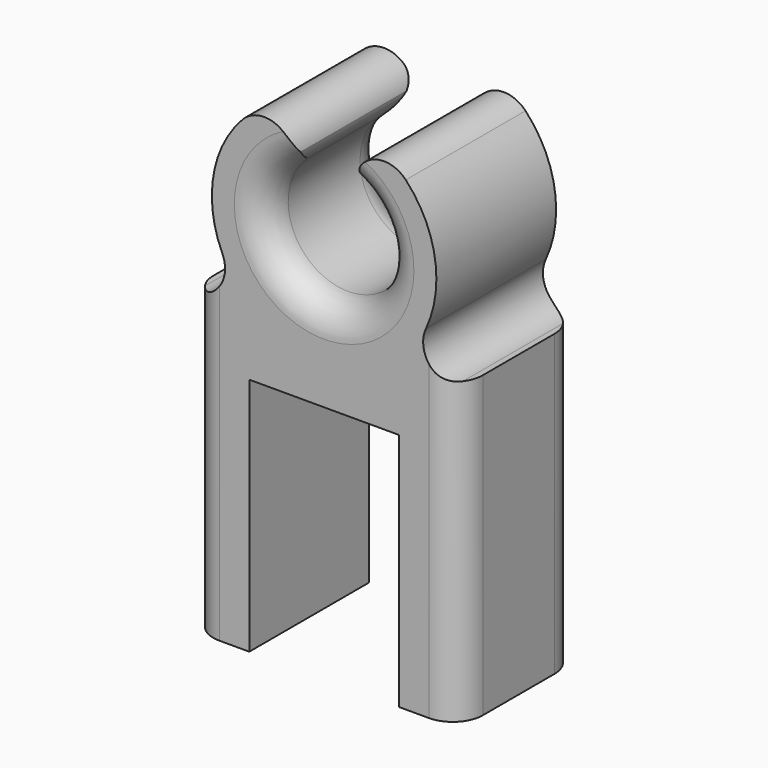
from build123d import *

# Parameters (mm, degrees)
F1_DEPTH    = 5
F2_R        = 7.5
F2_R_2      = 4
F3_DEPTH    = 5
F4_W        = 4
F4_H        = 10
F5_DEPTH    = 5.7
F6_T1_DEPTH = 10
F6_T3_DEPTH = 30.1640895286
F6_T5_DEPTH = 15.0401716993
F7_R        = 2
F8_T2_ANGLE = 359.64
F8_T4_ANGLE = 359.64


# Not quite as in the source:
# - a fillet or chamfer that OpenCascade refuses, or shapes differently, is made with other operations: its cross-section is extruded or revolved along the edge and cut away or added


with BuildPart() as f1:
    # F0 (on Front) → F1 (new body, symmetric)
    with BuildSketch(Plane.XZ):
        Polygon((-4, 0), (0, 0), (0, 16), (10, 16), (10, 0), (14, 0), (14, 20), (-4, 20), align=None)
    extrude(amount=F1_DEPTH, both=True)

    # F2 (on Front) → F3 (join, symmetric)
    with BuildSketch(Plane.XZ):
        with Locations((5, 26)):
            Circle(F2_R)
        with Locations((5, 26)):
            Circle(F2_R_2, mode=Mode.SUBTRACT)
    extrude(amount=F3_DEPTH, both=True)

    # F4 (on Front) → F5 (cut, symmetric)
    with BuildSketch(Plane.XZ):
        with Locations((5, 31.8401088891)):
            Rectangle(F4_W, F4_H)
    extrude(amount=F5_DEPTH, both=True, mode=Mode.SUBTRACT)

    # F6: fillet of radius 2 on 6 edges, made by hand

    # F6_s2 → F6_t1 (join)
    with BuildSketch(Plane.XZ.offset(-5)):
        with BuildLine():
            ThreePointArc((-3.6168439698, 20), (-1.930989509, 20.9239448263), (-1.8027715551, 22.8421052632))
            ThreePointArc((-1.8027715551, 22.8421052632), (-0.8273108539, 21.2785120765), (0.5, 20))
            Line((0.5, 20), (-3.6168439698, 20))
        make_face()
        with BuildLine():
            ThreePointArc((11.8027715551, 22.8421052632), (11.930989509, 20.9239448263), (13.6168439698, 20))
            Line((13.6168439698, 20), (9.5, 20))
            ThreePointArc((9.5, 20), (10.8273108539, 21.2785120765), (11.8027715551, 22.8421052632))
        make_face()
    extrude(amount=F6_T1_DEPTH)

    # F6_s4 → F6_t3 (cut)
    with BuildSketch(Plane.XZ.offset(-15.0820447643)):
        with BuildLine():
            ThreePointArc((10.4545454545, 31.1476143877), (8.2614510541, 31.6335579722), (7, 29.7749172176))
            Line((7, 29.7749172176), (7, 33.2284161474))
            ThreePointArc((7, 33.2284161474), (8.869753994, 32.4245625552), (10.4545454545, 31.1476143877))
        make_face()
        with BuildLine():
            ThreePointArc((3, 29.7749172176), (1.7385489459, 31.6335579722), (-0.4545454545, 31.1476143877))
            ThreePointArc((-0.4545454545, 31.1476143877), (1.130246006, 32.4245625552), (3, 33.2284161474))
            Line((3, 33.2284161474), (3, 29.7749172176))
        make_face()
    extrude(amount=F6_T3_DEPTH, mode=Mode.SUBTRACT)

    # F6_s6 → F6_t5 (cut)
    with BuildSketch(Plane.XZ.offset(-7.5200858497)):
        with BuildLine():
            ThreePointArc((7, 30.472135955), (7.1742581416, 29.6556393741), (7.6666666667, 28.98142397))
            ThreePointArc((7.6666666667, 28.98142397), (7.3457810792, 29.2399554207), (7, 29.4641016151))
            Line((7, 29.4641016151), (7, 30.472135955))
        make_face()
        with BuildLine():
            ThreePointArc((2.3333333333, 28.98142397), (2.8257418584, 29.6556393741), (3, 30.472135955))
            Line((3, 30.472135955), (3, 29.4641016151))
            ThreePointArc((3, 29.4641016151), (2.6542189208, 29.2399554207), (2.3333333333, 28.98142397))
        make_face()
    extrude(amount=F6_T5_DEPTH, mode=Mode.SUBTRACT)

    # F7
    f7_edges = [f1.edges().sort_by_distance(p)[0] for p in [
        (-4, -5, 10),
        (14, -5, 10),
        (14, 5, 10),
        (-4, 5, 10),
    ]]
    fillet(f7_edges, radius=F7_R)

    # F8: fillet of radius 2 on 2 edges, made by hand

    # F8_s1 → F8_t2 (revolve, cut)
    with BuildSketch(Plane(origin=(4.9182697806, 0, -0.015451251), x_dir=(0, 1, 0), z_dir=(-0.9999950652, 0, 0.0031415875))):
        with BuildLine():
            ThreePointArc((-5, -32.0155796327), (-4.4142135624, -30.6013660703), (-3, -30.0155796327))
            Line((-3, -30.0155796327), (-5, -30.0155796327))
            Line((-5, -30.0155796327), (-5, -32.0155796327))
        make_face()
    revolve(axis=Axis((5, -5, 26), (0, 1, 0)), revolution_arc=F8_T2_ANGLE, mode=Mode.SUBTRACT)

    # F8_s3 → F8_t4 (revolve, cut)
    with BuildSketch(Plane(origin=(5.0816315237, 0, 0.0159644688), x_dir=(0, 1, 0), z_dir=(0.9999950652, 0, 0.0031415875))):
        with BuildLine():
            ThreePointArc((5, 31.9841637578), (4.4142135624, 30.5699501954), (3, 29.9841637578))
            Line((3, 29.9841637578), (5, 29.9841637578))
            Line((5, 29.9841637578), (5, 31.9841637578))
        make_face()
    revolve(axis=Axis((5, 5, 26), (0, -1, 0)), revolution_arc=F8_T4_ANGLE, mode=Mode.SUBTRACT)


solid = f1.part
